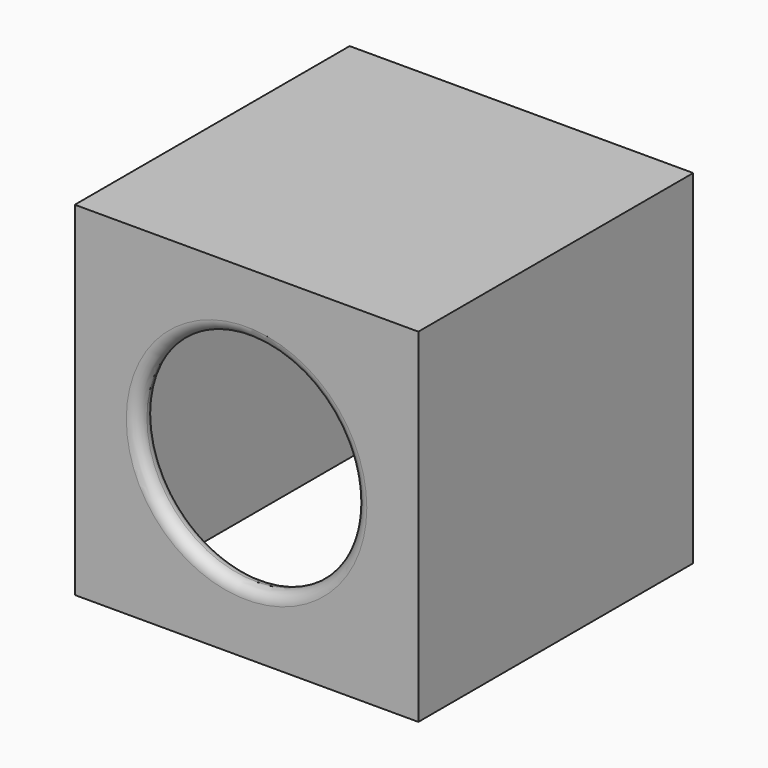
from build123d import *

# Parameters (mm, degrees)
F0_W     = 38.1
F0_H     = 38.1
F1_DEPTH = 38.1
F2_W     = 33.02
F2_H     = 33.02
F3_DEPTH = 35.56
F4_R     = 2.54
F5_R     = 12.065
F6_DEPTH = 38.101
F7_R     = 1.26999


# Not quite as in the source:
# - a fillet or chamfer is up to 0.001 mm smaller than in the source, because OpenCascade refuses the exact size


with BuildPart() as f1:
    # F0 (on Top) → F1 (new body)
    with BuildSketch(Plane.XY):
        with Locations((19.05, -19.05)):
            Rectangle(F0_W, F0_H)
    extrude(amount=F1_DEPTH)

    # F2 (on face) → F3 (cut)
    with BuildSketch(Plane(origin=(0, 0, 0), x_dir=(1, 0, 0), z_dir=(0, 0, -1))):
        with Locations((19.05, 19.05)):
            Rectangle(F2_W, F2_H)
    extrude(amount=-F3_DEPTH, mode=Mode.SUBTRACT)

    # F4
    f4_edges = [f1.edges().sort_by_distance(p)[0] for p in [
        (19.05, -35.56, 35.56),
        (2.54, -19.05, 35.56),
        (35.56, -19.05, 35.56),
        (19.05, -2.54, 35.56),
    ]]
    fillet(f4_edges, radius=F4_R)

    # F5 (on face) → F6 (cut, through all)
    with BuildSketch(Plane(origin=(0, 0, 0), x_dir=(-1, 0, 0), z_dir=(0, 1, 0))):
        with Locations((-19.05, 19.05)):
            Circle(F5_R)
    extrude(amount=-F6_DEPTH, mode=Mode.SUBTRACT)

    # F7 (radius 1.27 in the source; OpenCascade refuses exactly that, so slightly less here)
    f7_edges = [f1.edges().sort_by_distance(p)[0] for p in [
        (31.115, 0, 19.05),
        (31.115, -2.54, 19.05),
        (31.115, -35.56, 19.05),
        (31.115, -38.1, 19.05),
    ]]
    fillet(f7_edges, radius=F7_R)


solid = f1.part
